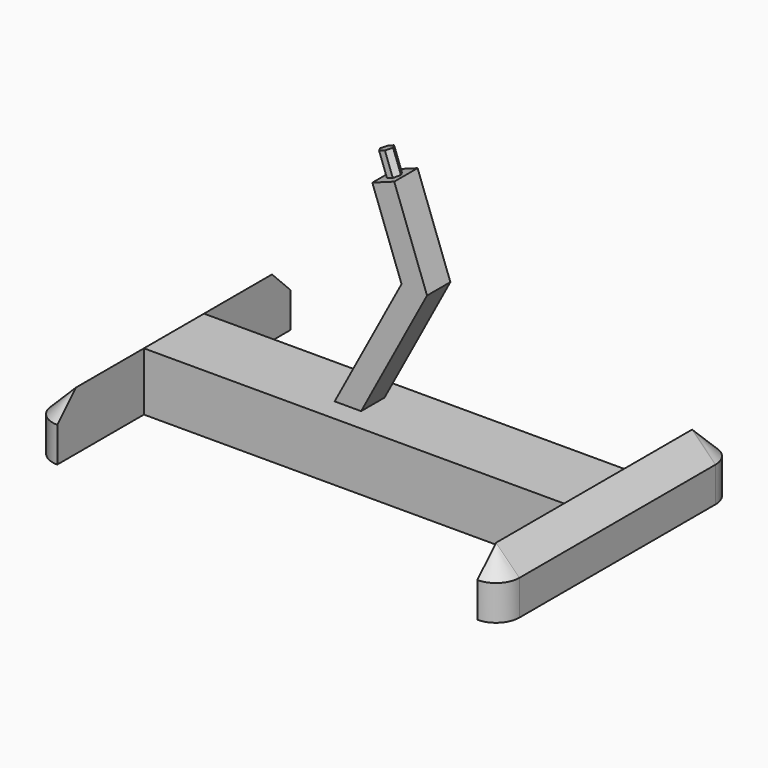
from build123d import *

# Parameters (mm, degrees)
F1_DEPTH     = 31.75
F2_DEPTH     = 3.175
F3_R         = 5.08
F4_SIZE      = 5.08
F6_DEPTH     = 5
F7_W         = 91.44
F7_H         = 18.495
F7_H_2       = 5.2874810565
F8_DEPTH     = 12.701
F9_T         = 5.08
F9_T3_DEPTH  = 22.86
F9_T5_DEPTH  = 16.51
F9_T7_DEPTH  = 15.9213350007
F9_T9_DEPTH  = 11.66
F9_T11_DEPTH = 11.5016876048
F9_T13_DEPTH = 11.66
F9_T15_DEPTH = 11.66
F9_T17_DEPTH = 11.5016876048
F9_T19_DEPTH = 11.66


# Not quite as in the source:
# - a shell that OpenCascade refuses in one call is made with other operations: the cavity is built on its own and cut out


with BuildPart() as f1:
    # F0 (on Front) → F1 (new body, symmetric)
    with BuildSketch(Plane.XZ):
        Polygon((50.8, -6.35), (50.8, 6.35), (-2.4423953146, 6.35), (-8.2037303153, 6.35), (-50.8, 6.35), (-50.8, -6.35), align=None)
    extrude(amount=F1_DEPTH, both=True)

    # F0 (on Front) → F2 (join, symmetric)
    with BuildSketch(Plane.XZ):
        Polygon((-8.2037303153, 6.35), (-2.4423953146, 6.35), (11.905341187, 33.1679385818), (4.7710500911, 52.6789357495), (0, 50.9343780577), (6.3533243835, 33.5591837482), align=None)
    extrude(amount=F2_DEPTH, both=True)

    # F3
    f3_edges = [f1.edges().sort_by_distance(p)[0] for p in [
        (-50.8, -31.75, 0),
        (50.8, -31.75, 0),
        (50.8, 31.75, 0),
        (-50.8, 31.75, 0),
    ]]
    fillet(f3_edges, radius=F3_R)

    # F4
    f4_edges = [f1.edges().sort_by_distance(p)[0] for p in [
        (50.8, 0, 6.35),
    ]]
    chamfer(f4_edges, length=F4_SIZE)

    # F5 (on face) → F6 (join)
    with BuildSketch(Plane(origin=(-16.4279316214, 0, 44.9274248875), x_dir=(0.9391830795, 0, 0.3434168651), z_dir=(-0.3434168651, 0, 0.9391830795))):
        Polygon((20.5937571299, 1.25), (19.2520695251, 1.25), (18.4229133275, 0), (19.2520695251, -1.25), (20.5937571299, -1.25), (21.4229133275, 0), align=None)
    extrude(amount=F6_DEPTH)

    # F7 (on face) → F8 (cut, through all)
    with BuildSketch(Plane.XY.offset(6.35)):
        with Locations((0, -17.4225)):
            Rectangle(F7_W, F7_H)
        with Locations((0, 17.4225)):
            Rectangle(F7_W, F7_H)
        with Locations((0, -29.3137405282)):
            Rectangle(F7_W, F7_H_2)
        with Locations((0, 29.3137405282)):
            Rectangle(F7_W, F7_H_2)
    extrude(amount=-F8_DEPTH, mode=Mode.SUBTRACT)

    # F9: shell of thickness 5.08, made by hand


with BuildPart() as f9_core1:
    # F9_t2: copy of F1
    add(f1.part)

    # the walls: a layer under each face that stays
    f9_faces = [f9_core1.faces().sort_by_distance(p)[0] for p in [
        (50.8, 0, -2.54),
        (48.26, 0, 3.81),
        (47.5160512242, 28.4660512242, 3.81),
        (45.72, 19.9625, 0),
        (0, 0, 6.35),
        (45.72, -19.9625, 0),
        (47.5160512242, -28.4660512242, 3.81),
        (-50.8, 0, -2.54),
        (-45.72, -19.9625, 0),
        (0, -8.175, 0),
        (0, 8.175, 0),
        (-45.72, 19.9625, 0),
        (-48.26, 0, 3.81),
        (-0.9252029659, 0, 19.9545918741),
        (8.55382927, 3.175, 29.5144678748),
        (8.55382927, -3.175, 29.5144678748),
        (4.7314729362, 0, 19.7589692909),
        (-47.5160512242, 28.4660512242, 3.81),
        (-47.5160512242, -28.4660512242, 3.81),
        (3.1766621917, 0, 42.246780903),
        (8.3381956391, 0, 42.9234371656),
        (3.975875076, 2.1166666667, 52.3881761342),
        (2.444199191, 0.625, 54.4899992105),
        (1.4247893073, 1.25, 54.1172470239),
        (0.4053794236, 0.625, 53.7444948373),
        (0.4053794236, -0.625, 53.7444948373),
        (1.4247893073, -1.25, 54.1172470239),
        (2.444199191, -0.625, 54.4899992105),
        (0.5662471447, 0, 56.4652047226),
    ]]
    thicken(f9_faces, amount=-F9_T, mode=Mode.SUBTRACT)

    # F9_s4 → F9_t3 (cut)
    with BuildSketch(Plane.XY.offset(-11.43)):
        Polygon((45.6692, 8.2258), (50.8, 8.175), (50.8, 3.095), (45.72, 3.095), align=None)
        Polygon((45.6692, -8.2258), (50.8, -8.175), (50.8, -3.095), (45.72, -3.095), align=None)
        Polygon((-45.6692, -8.2258), (-50.8, -8.175), (-50.8, -3.095), (-45.72, -3.095), align=None)
        Polygon((-45.6692, 8.2258), (-45.72, 3.095), (-50.8, 3.095), (-50.8, 8.175), align=None)
    extrude(amount=F9_T3_DEPTH, mode=Mode.SUBTRACT)

    # F9_s6 → F9_t5 (cut)
    with BuildSketch(Plane.XZ.offset(-8.255)):
        Polygon((-8.2485227119, 6.424764165), (-8.2037303153, 1.27), (-5.1602217701, 1.27), (-3.7244906507, 3.9535835029), align=None)
        Polygon((-2.3976029179, 6.376835835), (-2.4423953146, 1.27), (-10.9215566565, 1.27), (-6.9216349791, 8.7464164971), align=None)
        Polygon((6.2608214864, 33.5657023365), (10.832564048, 31.1627672512), (11.9053411319, 33.1679385857), (11.1243744273, 35.3037414227), align=None)
    extrude(amount=F9_T5_DEPTH, mode=Mode.SUBTRACT)

    # F9_s8 → F9_t7 (cut)
    with BuildSketch(Plane.YZ.offset(-13.2837303153)):
        Polygon((3.2258, 6.4008), (3.175, 1.27), (-1.905, 1.27), (-1.905, 6.35), align=None)
        Polygon((-3.2258, 6.4008), (-3.175, 1.27), (1.905, 1.27), (1.905, 6.35), align=None)
    extrude(amount=F9_T7_DEPTH, mode=Mode.SUBTRACT)

    # F9_s10 → F9_t9 (cut)
    with BuildSketch(Plane(origin=(8.7850864423, -14.1016340866, 3.2123096243), x_dir=(-0.8487666121, -0.5287676599, 0), z_dir=(-0.5191529807, 0.8333333333, -0.1898308147))):
        Polygon((-3.1675232496, 51.0265185517), (-4.6144586839, 46.1037076546), (0.2449508944, 44.6229853476), (1.7256732014, 49.4823949258), align=None)
    extrude(amount=F9_T9_DEPTH, mode=Mode.SUBTRACT)

    # F9_s12 → F9_t11 (cut)
    with BuildSketch(Plane(origin=(24.1123582833, 0, 8.8168011877), x_dir=(0, 1, 0), z_dir=(-0.9391830795, 0, -0.3434168651))):
        Polygon((1.3008, -47.8875060361), (1.25, -42.7567060361), (-3.83, -42.7567060361), (-3.83, -47.8367060361), align=None)
    extrude(amount=F9_T11_DEPTH, mode=Mode.SUBTRACT)

    # F9_s14 → F9_t13 (cut)
    with BuildSketch(Plane(origin=(8.7028980905, 13.9697070906, 3.1822570534), x_dir=(0.8487666121, -0.5287676599, 0), z_dir=(-0.5191529807, -0.8333333333, -0.1898308147))):
        Polygon((0.6788933364, 50.2682021828), (2.2230169623, 45.3750057318), (7.0824265406, 46.8557280388), (5.6017042336, 51.7151376171), align=None)
    extrude(amount=F9_T13_DEPTH, mode=Mode.SUBTRACT)

    # F9_s16 → F9_t15 (cut)
    with BuildSketch(Plane(origin=(2.6495743357, -4.253040424, 0.9688297542), x_dir=(0.8487666121, 0.5287676599, 0), z_dir=(0.5191529807, -0.8333333333, 0.1898308147))):
        Polygon((0.6788933364, 50.2682021828), (2.2230169623, 45.3750057318), (7.0824265406, 46.8557280388), (5.6017042336, 51.7151376171), align=None)
    extrude(amount=F9_T15_DEPTH, mode=Mode.SUBTRACT)

    # F9_s18 → F9_t17 (cut)
    with BuildSketch(Plane(origin=(13.3101678993, 0, 4.8669276876), x_dir=(0, 1, 0), z_dir=(0.9391830795, 0, 0.3434168651))):
        Polygon((-1.3008, 47.8875060361), (-1.25, 42.7567060361), (3.83, 42.7567060361), (3.83, 47.8367060361), align=None)
    extrude(amount=F9_T17_DEPTH, mode=Mode.SUBTRACT)

    # F9_s20 → F9_t19 (cut)
    with BuildSketch(Plane(origin=(2.7317626875, 4.38496742, 0.9988823252), x_dir=(-0.8487666121, 0.5287676599, 0), z_dir=(0.5191529807, 0.8333333333, 0.1898308147))):
        Polygon((-3.1675232496, 51.0265185517), (-4.6144586839, 46.1037076546), (0.2449508944, 44.6229853476), (1.7256732014, 49.4823949258), align=None)
    extrude(amount=F9_T19_DEPTH, mode=Mode.SUBTRACT)


with BuildPart() as f1_1:
    add(f1.part)

    # what is left inside the walls is the cavity
    f9_cavity = [f9_core1.part.solids().sort_by_distance(p)[0] for p in [
        (0, 3.0442, -3.81),
    ]]
    add(f9_cavity, mode=Mode.SUBTRACT)


solid = f1_1.part
